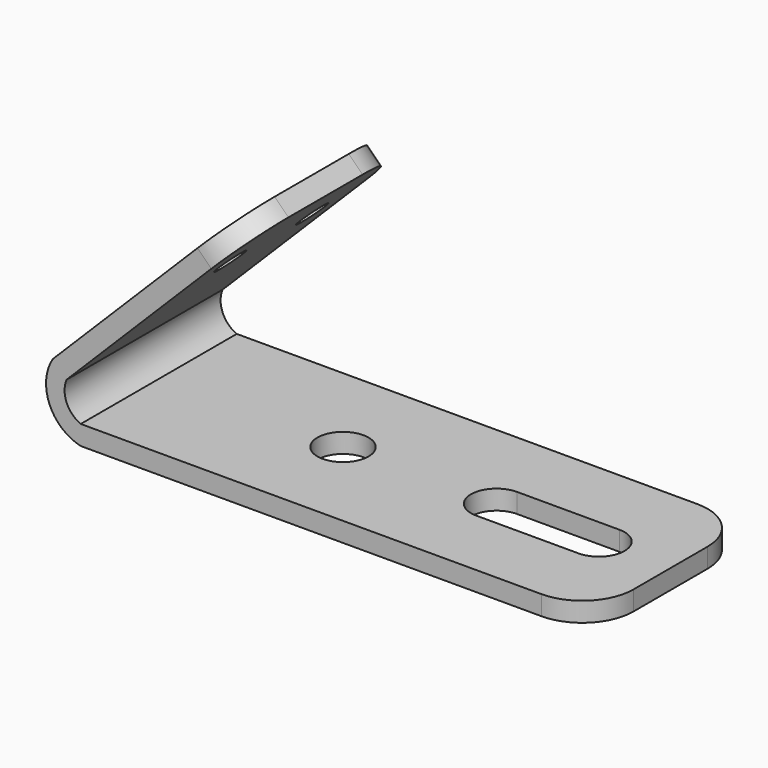
from build123d import *

# Parameters (mm, degrees)
F1_DEPTH  = 19.05
F2_R      = 5
F3_R      = 1.5
F4_DEPTH  = 10
F8_R      = 5
F9_R      = 2.5
F10_DEPTH = 25


with BuildPart() as f1:
    # F0 (on Front) → F1 (new body)
    with BuildSketch(Plane.XZ):
        with BuildLine():
            ThreePointArc((-2.7319921982, 6.5956126171), (-3.0542473294, 2.5985097523), (0, 0))
            Line((0, 0), (50, 0))
            Line((50, 0), (50, 1.9))
            Line((50, 1.9), (0, 1.9))
            ThreePointArc((0, 1.9), (-1.3800797918, 3.291972652), (-1.3884893139, 5.2521097328))
            Line((-1.3884893139, 5.2521097328), (16.2891802158, 22.9297792625))
            Line((16.2891802158, 22.9297792625), (14.9456773315, 24.2732821468))
            Line((14.9456773315, 24.2732821468), (-2.7319921982, 6.5956126171))
        make_face()
    extrude(amount=F1_DEPTH)

    # F2
    f2_edges = [f1.edges().sort_by_distance(p)[0] for p in [
        (15.617429, -19.05, 23.601531),
        (15.617429, 0, 23.601531),
    ]]
    fillet(f2_edges, radius=F2_R)

    # F3 (on face) → F4 (cut)
    with BuildSketch(Plane(origin=(-4.6638024076, 0, 4.6638024076), x_dir=(0, -1, 0), z_dir=(-0.7071067812, 0, 0.7071067812))):
        with Locations((14.55, 20.2319921982)):
            Circle(F3_R)
        with Locations((4.5, 20.2319921982)):
            Circle(F3_R)
    extrude(amount=-F4_DEPTH, mode=Mode.SUBTRACT)

    # F8
    f8_edges = [f1.edges().sort_by_distance(p)[0] for p in [
        (50, 0, 0.95),
        (50, -19.05, 0.95),
    ]]
    fillet(f8_edges, radius=F8_R)

    # F9 (on face) → F10 (cut)
    with BuildSketch(Plane.XY.offset(1.9)):
        with Locations((18, -9.525)):
            Circle(F9_R)
        with BuildLine():
            Line((33, -12.025), (43, -12.025))
            ThreePointArc((43, -12.025), (45.5, -9.525), (43, -7.025))
            Line((43, -7.025), (33, -7.025))
            ThreePointArc((33, -7.025), (30.5, -9.525), (33, -12.025))
        make_face()
    extrude(amount=-F10_DEPTH, mode=Mode.SUBTRACT)


solid = f1.part
